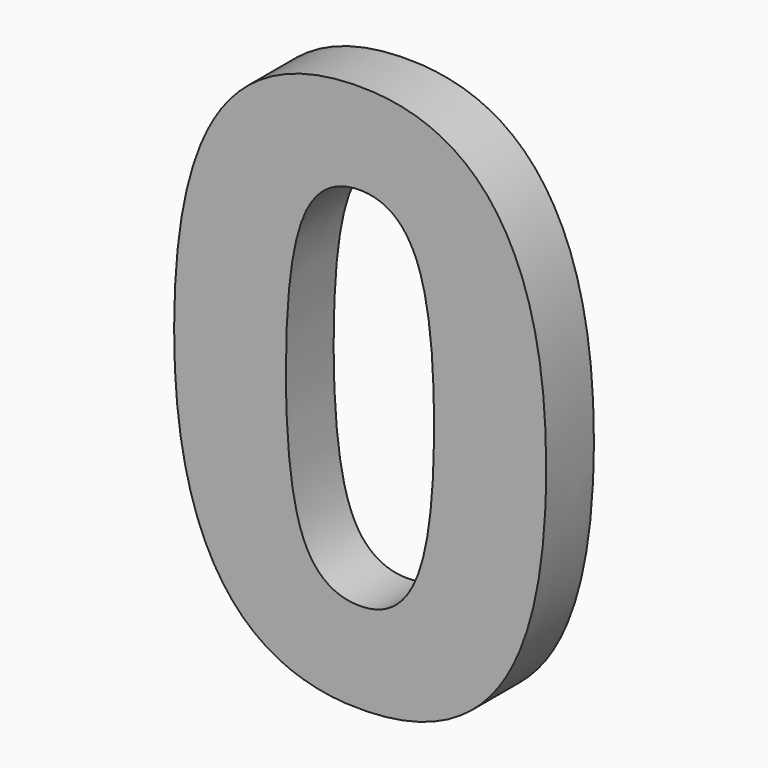
from build123d import *

# Parameters (mm, degrees)
F0_TEXT_SIZE = 62.5
F1_DEPTH     = 5


# Not quite as in the source:
# - Text() gives the source's letters only with a copy of the font that has no kerning and outlines rounded to 1/6400 em; it was checked with that copy


with BuildPart() as f1:
    # F0 (on Front) → F1 (new body)
    with BuildSketch(Plane.XZ):
        with Locations((-57.2368411395, 9.8684205698)):
            Text('0', F0_TEXT_SIZE, font='Open Sans', font_style=FontStyle.BOLD, text_align=(TextAlign.LEFT, TextAlign.BOTTOM))
    extrude(amount=F1_DEPTH)


solid = f1.part
